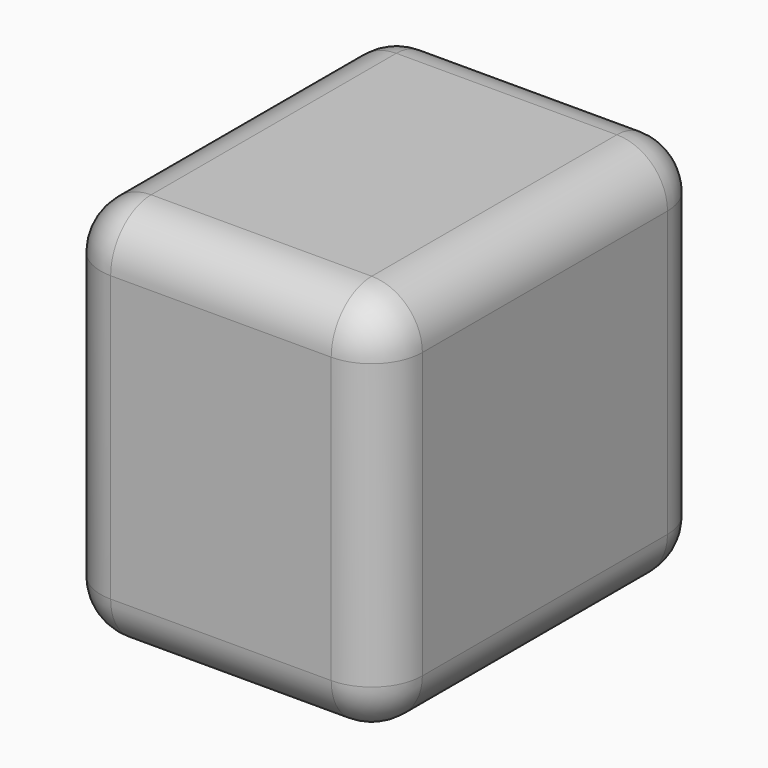
from build123d import *

# Parameters (mm, degrees)
F0_W         = 31.7708179355
F0_H         = 27.5444276631
F1_DEPTH     = 38.1
F2_DEPTH     = 12.7
F3_R         = 5
F4_T1_DEPTH  = 28.1
F4_S5_W      = 5
F4_S5_H      = 5
F4_T6_DEPTH  = 5
F4_S11_W     = 5
F4_S11_H     = 5
F4_T12_DEPTH = 5


# Not quite as in the source:
# - a fillet or chamfer that OpenCascade refuses, or shapes differently, is made with other operations: its cross-section is extruded or revolved along the edge and cut away or added


with BuildPart() as f1:
    # F0 (on Top) → F1 (new body)
    with BuildSketch(Plane.XY):
        with Locations((15.8854089677, -13.7722138315)):
            Rectangle(F0_W, F0_H)
    extrude(amount=F1_DEPTH)

    # F2 (add): a face of the model
    f2_faces = [f1.faces().sort_by_distance(p)[0] for p in [
        (15.8854089677, -27.5444276631, 19.05),
    ]]
    extrude(f2_faces, amount=F2_DEPTH)

    # F3
    f3_edges = [f1.edges().sort_by_distance(p)[0] for p in [
        (0, -40.244428, 19.05),
        (0, -20.122214, 38.1),
        (31.770818, -20.122214, 0),
        (31.770818, -20.122214, 38.1),
        (31.770818, -40.244428, 19.05),
        (15.885409, 0, 38.1),
        (15.885409, -40.244428, 0),
        (0, -20.122214, 0),
        (15.885409, -40.244428, 38.1),
        (15.885409, 0, 0),
        (0, 0, 19.05),
    ]]
    fillet(f3_edges, radius=F3_R)

    # F4: fillet of radius 5 on 1 edges, made by hand

    # F4_s2 → F4_t1 (cut)
    with BuildSketch(Plane.XY.offset(5)):
        with BuildLine():
            ThreePointArc((26.7708179355, 0), (30.3063518414, -1.4644660941), (31.7708179355, -5))
            Line((31.7708179355, -5), (31.7708179355, 0))
            Line((31.7708179355, 0), (26.7708179355, 0))
        make_face()
    extrude(amount=F4_T1_DEPTH, mode=Mode.SUBTRACT)


with BuildPart() as f4_tool4:
    # F4_s5 → F4_t6 (new body)
    with BuildSketch(Plane.XZ.offset(5)):
        with Locations((29.2708179355, 2.5)):
            Rectangle(F4_S5_W, F4_S5_H)
    extrude(amount=-F4_T6_DEPTH)

    # F4_s7 → F4_t8 (revolve, cut)
    with BuildSketch(Plane(origin=(26.7708179355, -5, 5), x_dir=(-0.7071067812, 0, 0.7071067812), z_dir=(-0.7071067812, 0, -0.7071067812))):
        with BuildLine():
            ThreePointArc((0, -5), (5, 0), (0, 5))
            Line((0, 5), (0, -5))
        make_face()
    revolve(axis=Axis((26.7708179355, -5, 5), (0, 1, 0)), mode=Mode.SUBTRACT)


with BuildPart() as f1_1:
    add(f1.part)

    # F4_t3: cut F4_tool4
    add(f4_tool4.part, mode=Mode.SUBTRACT)


with BuildPart() as f4_tool10:
    # F4_s11 → F4_t12 (new body)
    with BuildSketch(Plane.XZ.offset(5)):
        with Locations((29.2708179355, 35.6)):
            Rectangle(F4_S11_W, F4_S11_H)
    extrude(amount=-F4_T12_DEPTH)

    # F4_s13 → F4_t14 (revolve, cut)
    with BuildSketch(Plane(origin=(26.7708179355, -5, 33.1), x_dir=(-0.7071067812, 0, -0.7071067812), z_dir=(0.7071067812, 0, -0.7071067812))):
        with BuildLine():
            ThreePointArc((0, -5), (5, 0), (0, 5))
            Line((0, 5), (0, -5))
        make_face()
    revolve(axis=Axis((26.7708179355, -5, 33.1), (0, 1, 0)), mode=Mode.SUBTRACT)


with BuildPart() as f1_2:
    add(f1_1.part)

    # F4_t9: cut F4_tool10
    add(f4_tool10.part, mode=Mode.SUBTRACT)


solid = f1_2.part
